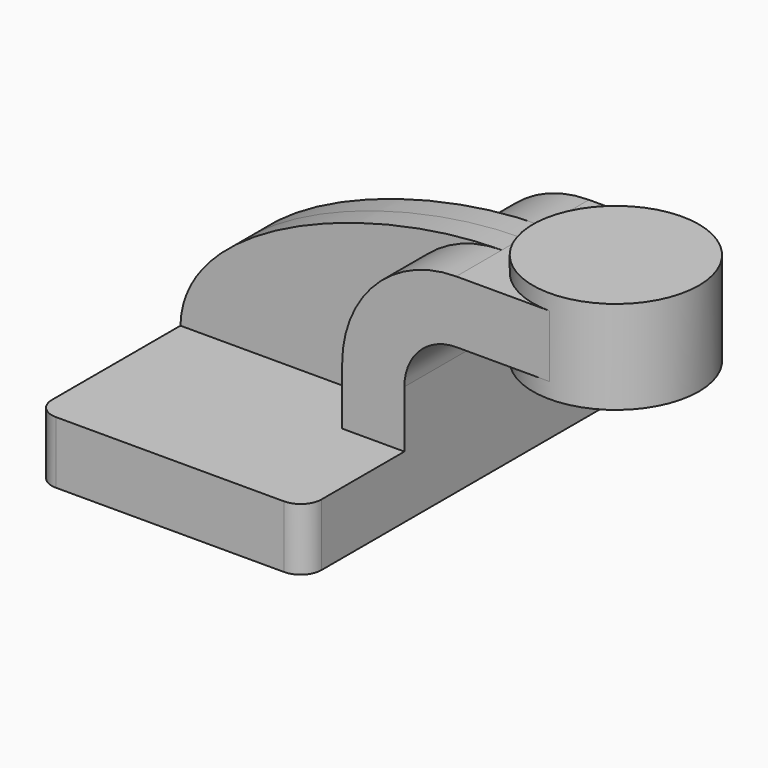
from build123d import *

# Parameters (mm, degrees)
F1_DEPTH = 63.5
F0_W     = 25.4
F0_H     = 19.05
F2_DEPTH = 25.4
F3_DEPTH = 7.9375
F5_R     = 6.35


# Not quite as in the source:
# - a feature names something its author has since deleted; it is built from what else it names


with BuildPart() as f1:
    # F0 (on Front) → F1 (new body, symmetric)
    with BuildSketch(Plane.XZ):
        Polygon((-41.275, 9.525), (-41.275, -9.525), (41.275, -9.525), (41.275, 9.525), (22.225, 9.525), align=None)
    extrude(amount=F1_DEPTH, both=True)

    # F0 (on Front) → F2 (join, symmetric)
    with BuildSketch(Plane.XZ):
        with Locations((73.025, 52.3875)):
            Rectangle(F0_W, F0_H)
        with BuildLine():
            Line((22.225, 9.525), (41.275, 9.525))
            Line((41.275, 9.525), (41.275, 26.9875))
            ThreePointArc((41.275, 26.9875), (45.9246798487, 38.2128201513), (57.15, 42.8625))
            Line((57.15, 42.8625), (60.325, 42.8625))
            Line((60.325, 42.8625), (60.325, 61.9125))
            Line((60.325, 61.9125), (57.15, 61.9125))
            ThreePointArc((57.15, 61.9125), (32.4542956671, 51.6832043329), (22.225, 26.9875))
            Line((22.225, 26.9875), (22.225, 9.525))
        make_face()
    extrude(amount=F2_DEPTH, both=True)

    # F0 (on Front) → F3 (join, symmetric)
    with BuildSketch(Plane.XZ):
        with BuildLine():
            add(Edge.make_bspline(
                [(-41.275, 9.525), (-40.6160876155, 40.568407625), (17.4937602133, 61.9470998645), (57.15, 61.9125)],
                knots=[0, 0, 0, 0, 111.4985685166, 111.4985685166, 111.4985685166, 111.4985685166], degree=3))
            Line((-41.275, 9.525), (22.225, 9.525))
            Line((22.225, 9.525), (22.225, 26.9875))
            ThreePointArc((22.225, 26.9875), (32.4542956671, 51.6832043329), (57.15, 61.9125))
        make_face()
    extrude(amount=F3_DEPTH, both=True)

    # F0 (on Front) → F4 (revolve)
    with BuildSketch(Plane.XZ):
        Polygon((85.725, 66.675), (85.725, 61.9125), (85.725, 42.8625), (85.725, 38.1), (111.125, 38.1), (111.125, 66.675), align=None)
    revolve(axis=Axis((85.725, 0, 52.3875), (0, 0, 1)))

    # F5
    f5_edges = [f1.edges().sort_by_distance(p)[0] for p in [
        (41.275, -63.5, 0),
        (-41.275, -63.5, 0),
        (41.275, 63.5, 0),
        (-41.275, 63.5, 0),
    ]]
    fillet(f5_edges, radius=F5_R)


solid = f1.part
